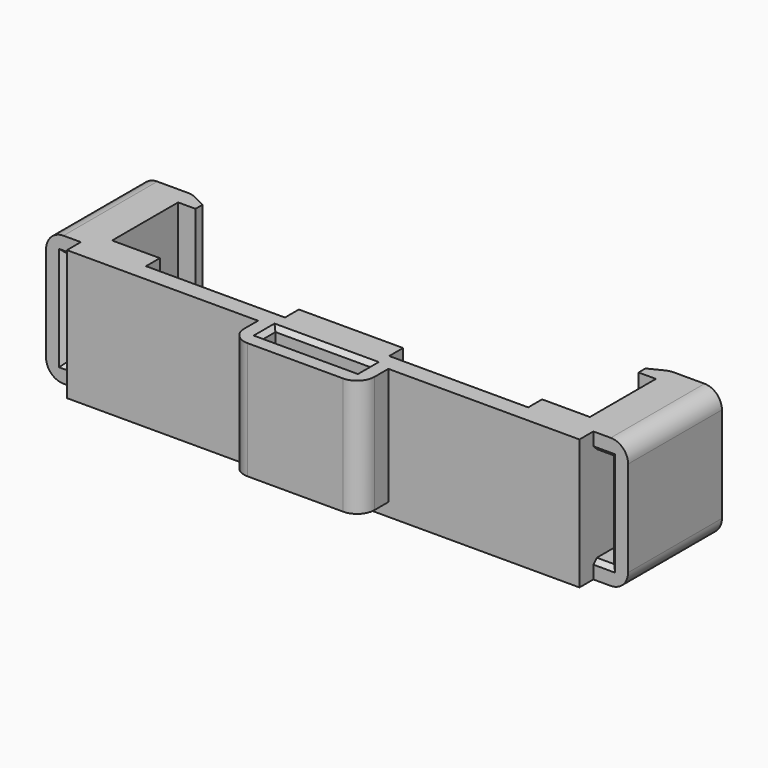
from build123d import *

# Parameters (mm, degrees)
F0_W     = 5.5
F0_H     = 2
F1_DEPTH = 15
F2_W     = 2
F2_H     = 11
F3_DEPTH = 13.501
F4_W     = 2
F4_H     = 2
F5_DEPTH = 13.5
F6_R     = 2
F7_SIZE  = 0.5


with BuildPart() as f1:
    # F0 (on Top) → F1 (new body)
    with BuildSketch(Plane.XY):
        Polygon((29.5, -1), (27.5, -1), (22, -1), (6, -1), (0, -1), (0, -3), (29.5, -3), align=None)
        with Locations((24.75, 0)):
            Rectangle(F0_W, F0_H)
        Polygon((27.5, 1), (27.5, -1), (29.5, -1), (29.5, 10.5), (27.5, 10.5), align=None)
        Polygon((29.5, 10.5), (29.5, -1), (33.5, -1), (33.5, 12.5), (29.5, 12.5), align=None)
        Polygon((0, -1), (6, -1), (6, 1), (-6, 1), (-6, -1), align=None)
        Polygon((25.5, 10.5), (27.5, 10.5), (29.5, 10.5), (29.5, 12.5), (27.5, 12.5), (25.5, 11.5), align=None)
        Polygon((0, -3), (0, -1), (-6, -1), (-22, -1), (-27.5, -1), (-29.5, -1), (-29.5, -3), align=None)
        with Locations((-24.75, 0)):
            Rectangle(F0_W, F0_H)
        Polygon((-29.5, 10.5), (-29.5, -1), (-27.5, -1), (-27.5, 1), (-27.5, 10.5), align=None)
        Polygon((-33.5, -1), (-29.5, -1), (-29.5, 10.5), (-29.5, 12.5), (-33.5, 12.5), align=None)
        Polygon((-29.5, 12.5), (-29.5, 10.5), (-27.5, 10.5), (-25.5, 10.5), (-25.5, 11.5), (-27.5, 12.5), align=None)
    extrude(amount=F1_DEPTH)

    # F2 (on face) → F3 (cut, through all)
    with BuildSketch(Plane.XZ.offset(1)):
        with Locations((-30.5, 7.5)):
            Rectangle(F2_W, F2_H)
        with Locations((30.5, 7.5)):
            Rectangle(F2_W, F2_H)
    extrude(amount=-F3_DEPTH, mode=Mode.SUBTRACT)

    # F4 (on face) → F5 (join)
    with BuildSketch(Plane.XY.offset(15)):
        with Locations((-6.5, -4)):
            Rectangle(F4_W, F4_H)
        Polygon((7.5, -7), (7.5, -3), (5.5, -3), (5.5, -5), (-5.5, -5), (-7.5, -5), (-7.5, -7), align=None)
    extrude(amount=-F5_DEPTH)

    # F6
    f6_edges = [f1.edges().sort_by_distance(p)[0] for p in [
        (33.5, 5.75, 15),
        (-33.5, 5.75, 15),
        (33.5, 5.75, 0),
        (-33.5, 5.75, 0),
        (-27.5, 12.5, 7.5),
        (27.5, 12.5, 7.5),
        (-7.5, -7, 8.25),
        (7.5, -7, 8.25),
    ]]
    fillet(f6_edges, radius=F6_R)

    # F7
    f7_edges = [f1.edges().sort_by_distance(p)[0] for p in [
        (-31.5, -1, 7.5),
        (-30.5, -1, 13),
        (-30.5, -1, 2),
        (31.5, -1, 7.5),
        (30.5, -1, 13),
        (30.5, -1, 2),
        (31.5, 12.5, 7.5),
        (30.5, 12.5, 2),
        (29.5, 12.5, 7.5),
        (30.5, 12.5, 13),
        (-30.5, 12.5, 2),
        (-29.5, 12.5, 7.5),
        (-31.5, 12.5, 7.5),
        (-30.5, 12.5, 13),
        (0, -3, 15),
        (-5.5, -4, 15),
        (0, -5, 15),
        (5.5, -4, 15),
    ]]
    chamfer(f7_edges, length=F7_SIZE)


solid = f1.part
